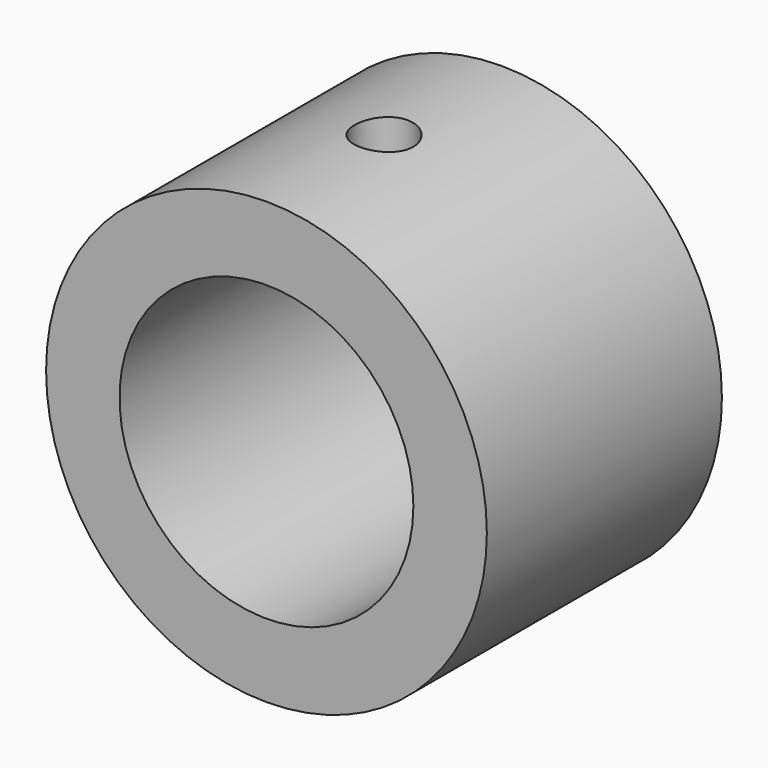
from build123d import *

# Parameters (mm, degrees)
F0_R     = 37.5
F0_R_2   = 25
F1_DEPTH = 25
F2_R     = 5
F3_DEPTH = 37.501


# Not quite as in the source:
# - a feature of the source that left no trace in its solid (it failed there, or was rolled back) is left out


with BuildPart() as f1:
    # F0 (on Front) → F1 (new body, symmetric)
    with BuildSketch(Plane.XZ):
        Circle(F0_R)
        Circle(F0_R_2, mode=Mode.SUBTRACT)
    extrude(amount=F1_DEPTH, both=True)

    # F2 (on Top) → F3 (cut, through all)
    with BuildSketch(Plane.XY):
        Circle(F2_R)
    extrude(amount=F3_DEPTH, mode=Mode.SUBTRACT)


solid = f1.part
